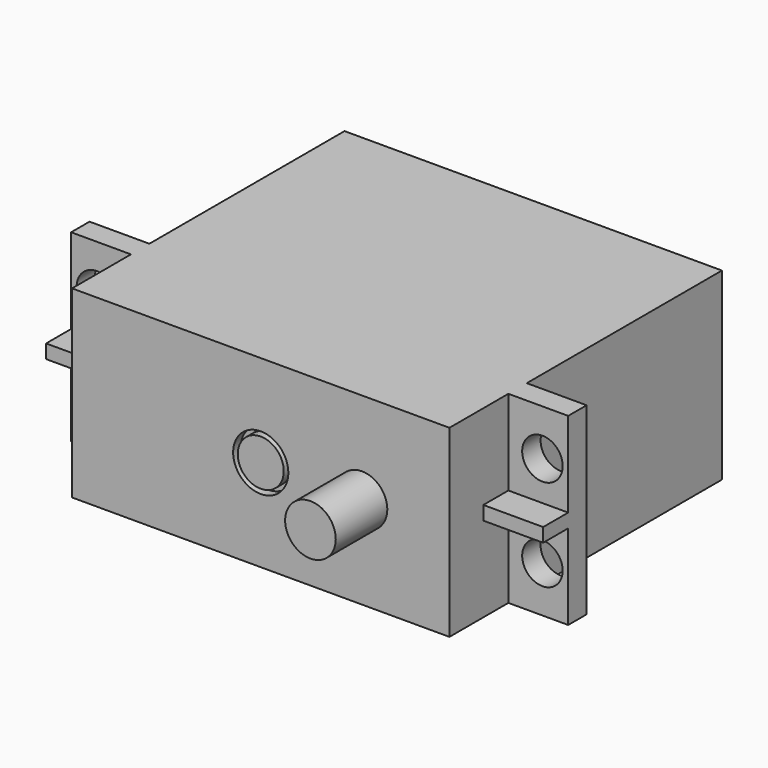
from build123d import *

# Parameters (mm, degrees)
F0_W      = 41
F0_H      = 20
F1_DEPTH  = 26.5
F2_W      = 6.5
F2_H      = 20
F2_R      = 2.2
F2_W_2    = 41
F3_DEPTH  = 2.5
F4_W      = 41
F4_H      = 20
F5_DEPTH  = 8
F6_W      = 6.5
F6_H      = 1.5
F7_DEPTH  = 3.4
F8_R      = 2.75
F9_DEPTH  = 7
F10_R     = 3
F10_R_2   = 2.5
F11_DEPTH = 1


# Not quite as in the source:
# - a pattern or mirror of a feature is missing from the dataset's text; its kind, count and spacing are read off the source's solid


with BuildPart() as f1:
    # F0 (on Front) → F1 (new body)
    with BuildSketch(Plane.XZ):
        Rectangle(F0_W, F0_H)
    extrude(amount=F1_DEPTH)

    # F2 (on face) → F3 (join)
    with BuildSketch(Plane.XZ.offset(26.5)):
        with Locations((-23.75, 0)):
            Rectangle(F2_W, F2_H)
        with Locations((-24.2, -5)):
            Circle(F2_R, mode=Mode.SUBTRACT)
        with Locations((-24.2, 5)):
            Circle(F2_R, mode=Mode.SUBTRACT)
        with Locations((23.75, 0)):
            Rectangle(F2_W, F2_H)
        with Locations((24.2, -5)):
            Circle(F2_R, mode=Mode.SUBTRACT)
        with Locations((24.2, 5)):
            Circle(F2_R, mode=Mode.SUBTRACT)
        Rectangle(F2_W_2, F2_H)
    extrude(amount=F3_DEPTH)

    # F4 (on face) → F5 (join)
    with BuildSketch(Plane.XZ.offset(29)):
        Rectangle(F4_W, F4_H)
    extrude(amount=F5_DEPTH)

    # F6 (on face) → F7 (join)
    with BuildSketch(Plane.XZ.offset(29)):
        with Locations((-23.75, 0)):
            Rectangle(F6_W, F6_H)
    f7 = extrude(amount=F7_DEPTH)

    # F7_copies: F7 across plane
    add(f7.mirror(Plane(origin=(0, 0, 0), x_dir=(0, 0, 1), z_dir=(1, 0, 0))))

    # F8 (on face) → F9 (join)
    with BuildSketch(Plane.XZ.offset(37)):
        with Locations((11, 0)):
            Circle(F8_R)
    extrude(amount=F9_DEPTH)

    # F10 (on face) → F11 (cut)
    with BuildSketch(Plane.XZ.offset(37)):
        Circle(F10_R)
        Circle(F10_R_2, mode=Mode.SUBTRACT)
    extrude(amount=-F11_DEPTH, mode=Mode.SUBTRACT)


solid = f1.part
